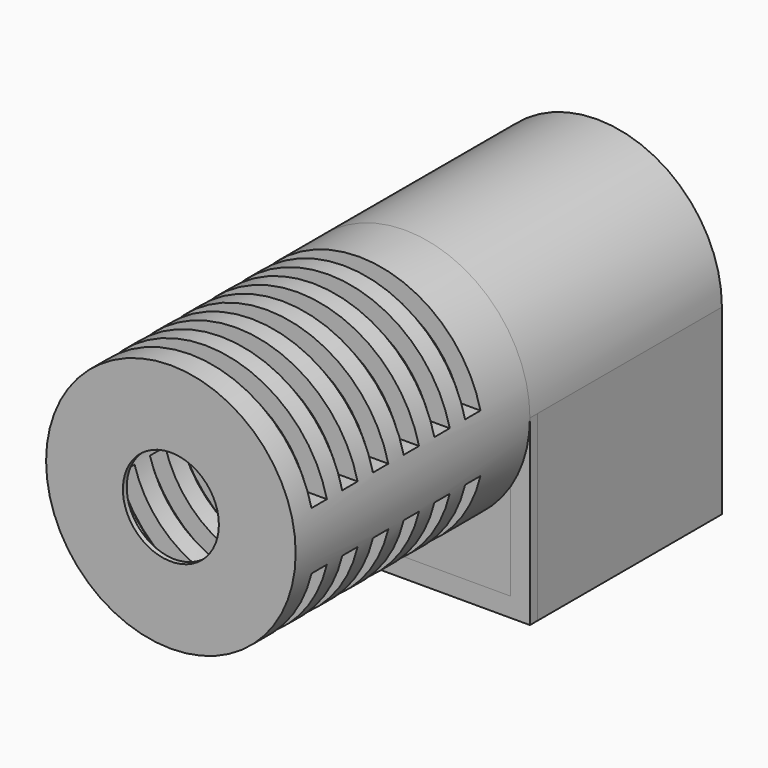
from build123d import *
from build123d import SkipClean  # not in build123d's __all__

# Parameters (mm, degrees)
F0_R      = 13
F0_R_2    = 11
F1_DEPTH  = 30
F2_R      = 13
F2_R_2    = 5
F3_DEPTH  = 0.5
F5_W      = 26
F5_H      = 2
F6_DEPTH  = 10
F8_W      = 26
F8_H      = 2
F9_DEPTH  = 10
F11_DEPTH = 25
F13_DEPTH = 1


with BuildPart() as f1:
    # F0 (on Front) → F1 (new body)
    with BuildSketch(Plane.XZ):
        Circle(F0_R)
        Circle(F0_R_2, mode=Mode.SUBTRACT)
    extrude(amount=-F1_DEPTH)

    # F2 (on Front) → F3 (join)
    with BuildSketch(Plane.XZ):
        Circle(F2_R)
        Circle(F2_R_2, mode=Mode.SUBTRACT)
    extrude(amount=F3_DEPTH)

    # F5 (on offset) → F6 (cut)
    with BuildSketch(Plane.XY.offset(13)):
        with Locations((-2.682e-07, 2.9999998622)):
            Rectangle(F5_W, F5_H)
        with Locations((-2.682e-07, 22.9999998622)):
            Rectangle(F5_W, F5_H)
        with Locations((-2.682e-07, 6.9999998622)):
            Rectangle(F5_W, F5_H)
        with Locations((-2.682e-07, 10.9999998622)):
            Rectangle(F5_W, F5_H)
        with Locations((-2.682e-07, 14.9999998622)):
            Rectangle(F5_W, F5_H)
        with Locations((-2.682e-07, 18.9999998622)):
            Rectangle(F5_W, F5_H)
    extrude(amount=-F6_DEPTH, mode=Mode.SUBTRACT)

    # F8 (on offset) → F9 (cut)
    with BuildSketch(Plane.XY.offset(-13)):
        with Locations((0, 3)):
            Rectangle(F8_W, F8_H)
        with Locations((0, 7)):
            Rectangle(F8_W, F8_H)
        with Locations((0, 11)):
            Rectangle(F8_W, F8_H)
        with Locations((0, 15)):
            Rectangle(F8_W, F8_H)
        with Locations((0, 19)):
            Rectangle(F8_W, F8_H)
        with Locations((0, 23)):
            Rectangle(F8_W, F8_H)
    extrude(amount=F9_DEPTH, mode=Mode.SUBTRACT)

    # F10 (on face) → F11 (join)
    with BuildSketch(Plane(origin=(0, 30, 0), x_dir=(-1, 0, 0), z_dir=(0, 1, 0))):
        with BuildLine():
            Line((11, 0), (11, -6.9282032303))
            ThreePointArc((11, -6.9282032303), (12.4899959968, -3.6055512755), (13, 0))
            ThreePointArc((13, 0), (0, 13), (-13, 0))
            ThreePointArc((-13, 0), (-12.4899959968, -3.6055512755), (-11, -6.9282032303))
            Line((-11, -6.9282032303), (-11, 0))
            ThreePointArc((-11, 0), (0, 11), (11, 0))
        make_face()
        with BuildLine():
            ThreePointArc((13, 0), (12.4899959968, -3.6055512755), (11, -6.9282032303))
            Line((11, -6.9282032303), (11, -17))
            Line((11, -17), (-11, -17))
            Line((-11, -17), (-11, -6.9282032303))
            ThreePointArc((-11, -6.9282032303), (-12.4899959968, -3.6055512755), (-13, 0))
            Line((-13, 0), (-13, -19))
            Line((-13, -19), (13, -19))
            Line((13, -19), (13, 0))
        make_face()
    with SkipClean():  # cleaning this boolean's faces spoils the solid; the shape is the same uncleaned
        extrude(amount=F11_DEPTH)

    # F12 (on face) → F13 (join)
    with BuildSketch(Plane(origin=(0, 30, 0), x_dir=(-1, 0, 0), z_dir=(0, 1, 0))):
        with BuildLine():
            Line((13, -19), (13, 0))
            ThreePointArc((13, 0), (12.4899959968, -3.6055512755), (11, -6.9282032303))
            ThreePointArc((11, -6.9282032303), (0, -13), (-11, -6.9282032303))
            ThreePointArc((-11, -6.9282032303), (-12.4899959968, -3.6055512755), (-13, 0))
            Line((-13, 0), (-13, -19))
            Line((-13, -19), (13, -19))
        make_face()
        with BuildLine():
            ThreePointArc((-11, -6.9282032303), (0, -13), (11, -6.9282032303))
            Line((11, -6.9282032303), (11, 0))
            ThreePointArc((11, 0), (0, -11), (-11, 0))
            Line((-11, 0), (-11, -6.9282032303))
        make_face()
    with SkipClean():  # cleaning this boolean's faces spoils the solid; the shape is the same uncleaned
        extrude(amount=F13_DEPTH)


solid = f1.part
